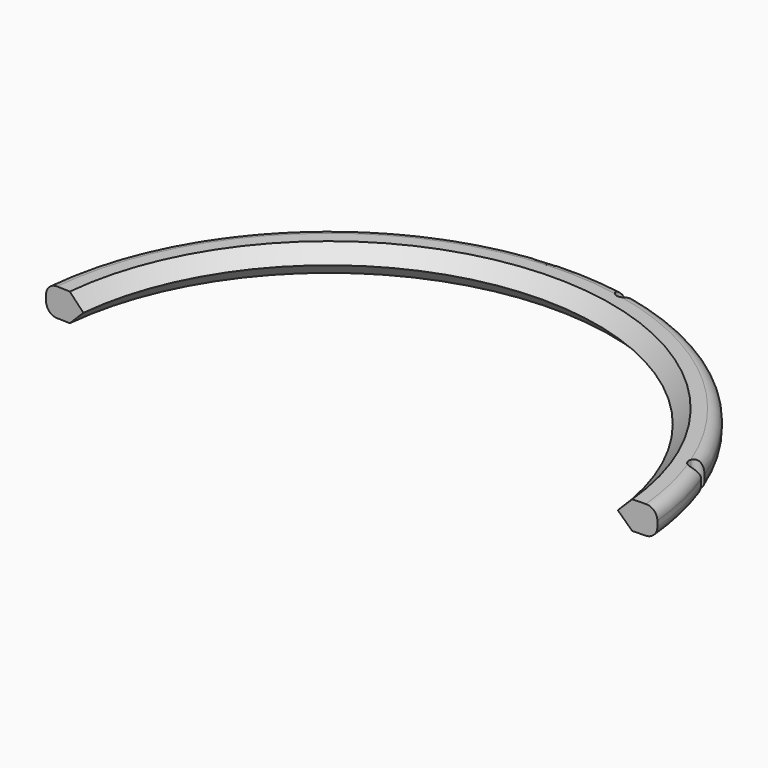
from build123d import *

# Parameters (mm, degrees)
F1_DEPTH  = 12.7
F2_R      = 5.08
F3_SIZE   = 6.34999
F7_DEPTH  = 25.4
F9_DEPTH  = 25.4
F6_R      = 3.175
F10_DEPTH = 25.4


# Not quite as in the source:
# - a fillet or chamfer is up to 0.001 mm smaller than in the source, because OpenCascade refuses the exact size


with BuildPart() as f1:
    # F0 (on Top) → F1 (new body)
    with BuildSketch(Plane.XY):
        with BuildLine():
            ThreePointArc((-85.1017062912, 39.9863691127), (36.5051433715, 149.8230416662), (158.1119930343, 39.9863691127))
            Line((158.1119930343, 39.9863691127), (175.5953490648, 40.6241259528))
            ThreePointArc((175.5953490648, 40.6241259528), (36.5051433715, 167.2855416662), (-102.5850623217, 40.6241259528))
            Line((-102.5850623217, 40.6241259528), (-85.1017062912, 39.9863691127))
        make_face()
    extrude(amount=F1_DEPTH)

    # F2
    f2_edges = [f1.edges().sort_by_distance(p)[0] for p in [
        (36.505143, 167.285542, 12.7),
        (36.505143, 167.285542, 0),
    ]]
    fillet(f2_edges, radius=F2_R)

    # F3 (size 6.35 in the source; OpenCascade refuses exactly that, so slightly less here)
    f3_edges = [f1.edges().sort_by_distance(p)[0] for p in [
        (36.505143, 149.823042, 12.7),
        (36.505143, 149.823042, 0),
    ]]
    chamfer(f3_edges, length=F3_SIZE)


with BuildPart() as f4_1:
    # F4: instance of F1
    add(f1.part.mirror(Plane.XY))


with BuildPart() as f1_1:
    add(f1.part)

    # F6 (on face) → F7 (cut)
    with BuildSketch(Plane.XY.offset(12.7)):
        with BuildLine():
            ThreePointArc((163.0583931619, 73.4856437086), (162.4024850501, 75.2552779595), (161.7218329639, 77.0155431585))
            ThreePointArc((161.7218329639, 77.0155431585), (161.8086296648, 75.0304207129), (163.0583931619, 73.4856437086))
        make_face()
    extrude(amount=-F7_DEPTH, mode=Mode.SUBTRACT)

    # F8 (on face) → F9 (cut)
    with BuildSketch(Plane.XY.offset(12.7)):
        with BuildLine():
            ThreePointArc((64.4226124591, 159.2789709622), (62.573664155, 159.6574032574), (60.7195923208, 160.0098780326))
            ThreePointArc((60.7195923208, 160.0098780326), (62.4506994343, 159.0344227782), (64.4226124591, 159.2789709622))
        make_face()
        with BuildLine():
            ThreePointArc((64.4226124591, 159.2789709622), (65.7478153328, 160.450521759), (66.2405230377, 162.1493251742))
            ThreePointArc((66.2405230377, 162.1493251742), (61.9182883246, 165.1098112007), (60.7195923208, 160.0098780326))
            ThreePointArc((60.7195923208, 160.0098780326), (62.573664155, 159.6574032574), (64.4226124591, 159.2789709622))
        make_face()
    extrude(amount=-F9_DEPTH, mode=Mode.SUBTRACT)

    # F6 (on face) → F10 (cut)
    with BuildSketch(Plane.XY.offset(12.7)):
        with Locations((164.7779065912, 76.1547069462)):
            Circle(F6_R)
    extrude(amount=-F10_DEPTH, mode=Mode.SUBTRACT)


solid = f1_1.part
